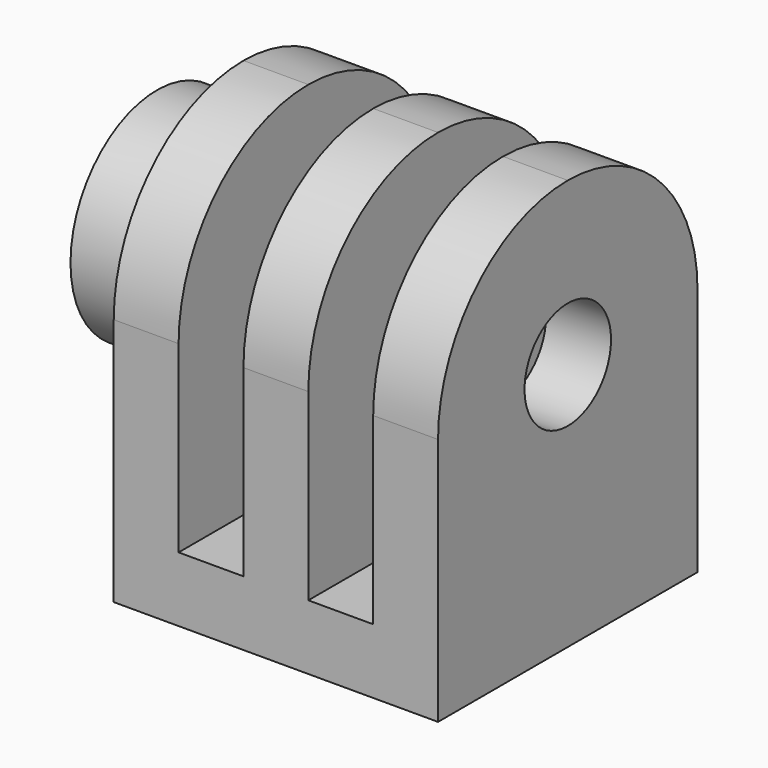
from build123d import *

# Parameters (mm, degrees)
F2_W     = 15
F2_H     = 15
F3_DEPTH = 3
F4_W     = 3
F4_H     = 15
F5_DEPTH = 16
F6_R     = 7.49999
F8_D     = 5
F7_R     = 5
F9_DEPTH = 4


# Not quite as in the source:
# - a fillet or chamfer is up to 0.001 mm smaller than in the source, because OpenCascade refuses the exact size


with BuildPart() as f3:
    # F2 (on Top) → F3 (new body)
    with BuildSketch(Plane.XY):
        Rectangle(F2_W, F2_H)
    extrude(amount=-F3_DEPTH)

    # F4 (on face) → F5 (join)
    with BuildSketch(Plane.XY):
        with Locations((-6, 0)):
            Rectangle(F4_W, F4_H)
        Rectangle(F4_W, F4_H)
        with Locations((6, 0)):
            Rectangle(F4_W, F4_H)
    extrude(amount=F5_DEPTH)

    # F6 (radius 7.5 in the source; OpenCascade refuses exactly that, so slightly less here)
    f6_edges = [f3.edges().sort_by_distance(p)[0] for p in [
        (-6, 7.5, 16),
        (0, 7.5, 16),
        (6, 7.5, 16),
        (-6, -7.5, 16),
        (0, -7.5, 16),
        (6, -7.5, 16),
    ]]
    fillet(f6_edges, radius=F6_R)

    # F8 (through all)
    with Locations(Plane(origin=(-7.5, 0, 0), x_dir=(0, -1, 0), z_dir=(-1, 0, 0))):
        with Locations((0, 8.5)):
            Hole(F8_D / 2)

    # F7 (on face) → F9 (join)
    with BuildSketch(Plane(origin=(-7.5, 0, 0), x_dir=(0, -1, 0), z_dir=(-1, 0, 0))):
        with Locations((0, 8.5)):
            Circle(F7_R)
        Polygon((-4.6188021535, 8.5), (-2.3094010768, 12.5), (2.3094010768, 12.5), (4.6188021535, 8.5), (2.3094010768, 4.5), (-2.3094010768, 4.5), align=None, mode=Mode.SUBTRACT)
    extrude(amount=F9_DEPTH)


solid = f3.part
